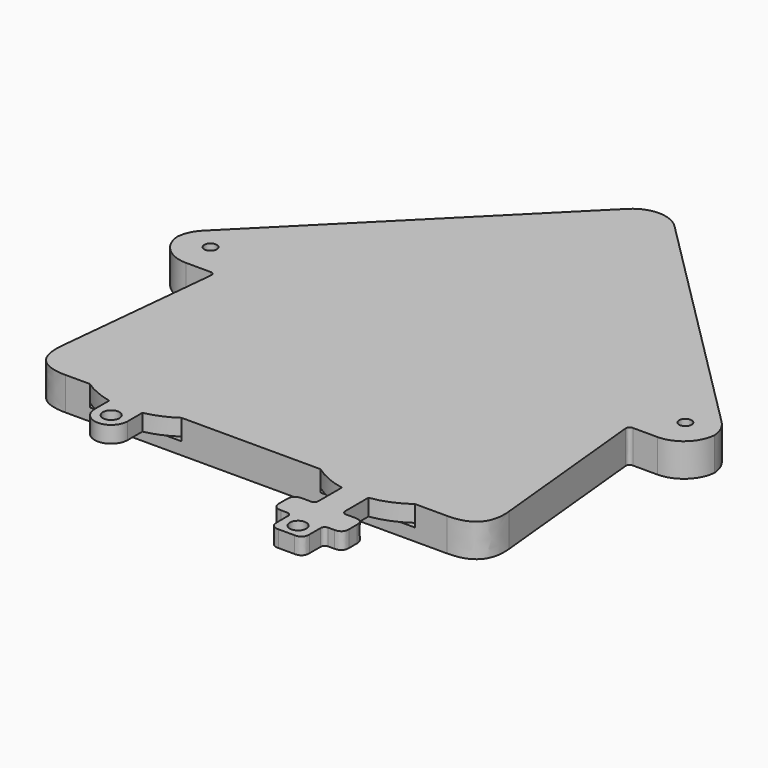
from build123d import *

# Parameters (mm, degrees)
F1_DEPTH    = 8
F2_T1_DEPTH = 24.5685424949
F2_T3_DEPTH = 48
F3_T1_DEPTH = 8
F4_T1_DEPTH = 52.1995024845
F5_R        = 13.5
F5_R_2      = 2
F6_DEPTH    = 5
F7_DEPTH    = 4
F8_T1_DEPTH = 14
F9_R        = 1
F10_R       = 1.5
F11_DEPTH   = 25


# Not quite as in the source:
# - a fillet or chamfer that OpenCascade refuses, or shapes differently, is made with other operations: its cross-section is extruded or revolved along the edge and cut away or added


with BuildPart() as f1:
    # F0 (on Top) → F1 (new body)
    with BuildSketch(Plane.XY):
        Polygon((65, 0), (0, 65), (-65, 0), (-65, -10), (-50, -10), (-55, -60), (0, -60), (55, -60), (50, -10), (65, -10), align=None)
    extrude(amount=F1_DEPTH)

    # F2: fillet of radius 8 on 5 edges, made by hand

    # F2_s2 → F2_t1 (cut)
    with BuildSketch(Plane.XY.offset(-8.2842712475)):
        with BuildLine():
            ThreePointArc((-65, -3.313708499), (-64.3910362601, -0.2522410401), (-62.6568542495, 2.3431457505))
            Line((-62.6568542495, 2.3431457505), (-65, 0))
            Line((-65, 0), (-65, -3.313708499))
        make_face()
        with BuildLine():
            ThreePointArc((62.6568542495, 2.3431457505), (64.3910362601, -0.2522410401), (65, -3.313708499))
            Line((65, -3.313708499), (65, 0))
            Line((65, 0), (62.6568542495, 2.3431457505))
        make_face()
    extrude(amount=F2_T1_DEPTH, mode=Mode.SUBTRACT)

    # F2_s4 → F2_t3 (cut)
    with BuildSketch(Plane.XY.offset(-20)):
        with BuildLine():
            ThreePointArc((5.6568542495, 59.3431457505), (0, 61.686291501), (-5.6568542495, 59.3431457505))
            Line((-5.6568542495, 59.3431457505), (0, 65))
            Line((0, 65), (5.6568542495, 59.3431457505))
        make_face()
        with BuildLine():
            ThreePointArc((57, -10), (62.6568542495, -7.6568542495), (65, -2))
            Line((65, -2), (65, -10))
            Line((65, -10), (57, -10))
        make_face()
        with BuildLine():
            ThreePointArc((-57, -10), (-62.6568542495, -7.6568542495), (-65, -2))
            Line((-65, -2), (-65, -10))
            Line((-65, -10), (-57, -10))
        make_face()
    extrude(amount=F2_T3_DEPTH, mode=Mode.SUBTRACT)

    # F3: fillet of radius 1 on 2 edges, made by hand

    # F3_s2 → F3_t1 (join)
    with BuildSketch(Plane.XY):
        with BuildLine():
            add(Edge.make_bspline(
                [(51.1049875621, -10), (50, -10), (50.1099503719, -11.099503719)],
                knots=[0, 0, 0, 1, 1, 1], degree=2, weights=[1, 1, 1]))
            Line((50.1099503719, -11.099503719), (50, -10))
            Line((50, -10), (51.1049875621, -10))
        make_face()
        with BuildLine():
            add(Edge.make_bspline(
                [(-50.1099503719, -11.099503719), (-50, -10), (-51.1049875621, -10)],
                knots=[0, 0, 0, 1, 1, 1], degree=2, weights=[1, 1, 1]))
            Line((-51.1049875621, -10), (-50, -10))
            Line((-50, -10), (-50.1099503719, -11.099503719))
        make_face()
    extrude(amount=F3_T1_DEPTH)

    # F4: fillet of radius 8 on 2 edges, made by hand

    # F4_s2 → F4_t1 (cut)
    with BuildSketch(Plane.XY.offset(-22.0997512422)):
        with BuildLine():
            add(Edge.make_bspline(
                [(-46.1600995031, -60), (-55, -60), (-54.1203970248, -51.2039702478)],
                knots=[0, 0, 0, 1, 1, 1], degree=2, weights=[1, 1, 1]))
            Line((-54.1203970248, -51.2039702478), (-55, -60))
            Line((-55, -60), (-46.1600995031, -60))
        make_face()
        with BuildLine():
            add(Edge.make_bspline(
                [(54.1203970248, -51.2039702478), (55, -60), (46.1600995031, -60)],
                knots=[0, 0, 0, 1, 1, 1], degree=2, weights=[1, 1, 1]))
            Line((46.1600995031, -60), (55, -60))
            Line((55, -60), (54.1203970248, -51.2039702478))
        make_face()
    extrude(amount=F4_T1_DEPTH, mode=Mode.SUBTRACT)

    # F5 (on face) → F6 (cut)
    with BuildSketch(Plane.XY.offset(8)):
        with BuildLine():
            Line((-8.4674237296, -19.0932191908), (-17.8053588669, -28.0791480434))
            ThreePointArc((-17.8053588669, -28.0791480434), (-45.0974523982, -32.7464944514), (-40.2098223871, -60))
            Line((-40.2098223871, -60), (-18.0631891992, -60))
            ThreePointArc((-18.0631891992, -60), (-11.8712274348, -53.0133159845), (-9.6365057932, -43.9490916266))
            ThreePointArc((-9.6365057932, -43.9490916266), (-10.5536669898, -38.0390914567), (-13.2188752299, -32.6850320897))
            Line((-13.2188752299, -32.6850320897), (-4.2390260021, -24.0298833133))
            Line((-4.2390260021, -24.0298833133), (-4.2390260021, -29.9932191908))
            Line((-4.2390260021, -29.9932191908), (1.8609739979, -29.9932191908))
            Line((1.8609739979, -29.9932191908), (1.8609739979, -12.9932191908))
            Line((1.8609739979, -12.9932191908), (-15.1390260021, -12.9932191908))
            Line((-15.1390260021, -12.9932191908), (-15.1390260021, -19.0932191908))
            Line((-15.1390260021, -19.0932191908), (-8.4674237296, -19.0932191908))
        make_face()
        with Locations((-29.1365057932, -43.9490916266)):
            Circle(F5_R, mode=Mode.SUBTRACT)
        with BuildLine():
            Line((-18.0631891992, -60), (-40.2098223871, -60))
            ThreePointArc((-40.2098223871, -60), (-36.8140065496, -61.8741015885), (-33.1144459271, -63.039036422))
            Line((-33.1144459271, -63.039036422), (-33.1144459271, -67.4490812726))
            ThreePointArc((-33.1144459271, -67.4490812726), (-29.1144459271, -71.4490812726), (-25.1144459271, -67.4490812726))
            Line((-25.1144459271, -67.4490812726), (-25.1144459271, -63.0297895812))
            ThreePointArc((-25.1144459271, -63.0297895812), (-21.4382914649, -61.8652155421), (-18.0631891992, -60))
        make_face()
        with Locations((-29.1144459271, -67.4490812726)):
            Circle(F5_R_2, mode=Mode.SUBTRACT)
        with BuildLine():
            Line((38.4021761528, -60), (15.5300545524, -60))
            ThreePointArc((15.5300545524, -60), (19.2758562864, -62.1250310842), (23.3967523072, -63.3760321733))
            Line((23.3967523072, -63.3760321733), (23.3967523072, -71.4671202268))
            Line((23.3967523072, -71.4671202268), (18.1967523072, -71.4671202268))
            Line((18.1967523072, -71.4671202268), (18.1967523072, -77.7814015746))
            Line((18.1967523072, -77.7814015746), (22.6967523072, -77.7814015746))
            Line((22.6967523072, -77.7814015746), (22.6967523072, -84.1620080173))
            Line((22.6967523072, -84.1620080173), (30.5967523072, -84.1620080173))
            Line((30.5967523072, -84.1620080173), (30.5967523072, -77.7814015746))
            Line((30.5967523072, -77.7814015746), (35.0967523072, -77.7814015746))
            Line((35.0967523072, -77.7814015746), (35.0967523072, -71.4671202268))
            Line((35.0967523072, -71.4671202268), (29.8967523072, -71.4671202268))
            Line((29.8967523072, -71.4671202268), (29.8967523072, -63.48401191))
            ThreePointArc((29.8967523072, -63.48401191), (34.357670388, -62.2502940054), (38.4021761528, -60))
        make_face()
        with Locations((26.6467523072, -80.6736797094)):
            Circle(F5_R_2, mode=Mode.SUBTRACT)
        with BuildLine():
            ThreePointArc((7.4678010834, -43.9490916266), (9.5407945482, -52.9581017828), (15.5300545524, -60))
            Line((15.5300545524, -60), (38.4021761528, -60))
            ThreePointArc((38.4021761528, -60), (35.9470895566, -26.8967619578), (7.4678010834, -43.9490916266))
        make_face()
        with BuildLine():
            ThreePointArc((40.4661153526, -44.2054910373), (26.8379098659, -57.7048822588), (13.4685504114, -43.9490916266))
            ThreePointArc((13.4685504114, -43.9490916266), (27.0943208393, -30.7060998157), (40.4661153526, -44.2054910373))
        make_face(mode=Mode.SUBTRACT)
    extrude(amount=-F6_DEPTH, mode=Mode.SUBTRACT)

    # F5 (on face) → F7 (join)
    with BuildSketch(Plane.XY.offset(8)):
        with BuildLine():
            Line((-8.4674237296, -19.0932191908), (-17.8053588669, -28.0791480434))
            ThreePointArc((-17.8053588669, -28.0791480434), (-46.9989205625, -36.1270625672), (-33.1144459271, -63.039036422))
            Line((-33.1144459271, -63.039036422), (-33.1144459271, -67.4490812726))
            ThreePointArc((-33.1144459271, -67.4490812726), (-29.1144459271, -71.4490812726), (-25.1144459271, -67.4490812726))
            Line((-25.1144459271, -67.4490812726), (-25.1144459271, -63.0297895812))
            ThreePointArc((-25.1144459271, -63.0297895812), (-13.99252733, -56.2336313537), (-9.6365057932, -43.9490916266))
            ThreePointArc((-9.6365057932, -43.9490916266), (-10.5536669898, -38.0390914567), (-13.2188752299, -32.6850320897))
            Line((-13.2188752299, -32.6850320897), (-4.2390260021, -24.0298833133))
            Line((-4.2390260021, -24.0298833133), (-4.2390260021, -29.9932191908))
            Line((-4.2390260021, -29.9932191908), (1.8609739979, -29.9932191908))
            Line((1.8609739979, -29.9932191908), (1.8609739979, -12.9932191908))
            Line((1.8609739979, -12.9932191908), (-15.1390260021, -12.9932191908))
            Line((-15.1390260021, -12.9932191908), (-15.1390260021, -19.0932191908))
            Line((-15.1390260021, -19.0932191908), (-8.4674237296, -19.0932191908))
        make_face()
        with Locations((-29.1144459271, -67.4490812726)):
            Circle(F5_R_2, mode=Mode.SUBTRACT)
        with Locations((-29.1365057932, -43.9490916266)):
            Circle(F5_R, mode=Mode.SUBTRACT)
        with BuildLine():
            ThreePointArc((29.8967523072, -63.48401191), (39.7733500471, -29.500908776), (7.4678010834, -43.9490916266))
            ThreePointArc((7.4678010834, -43.9490916266), (11.8869595763, -56.5695138889), (23.3967523072, -63.3760321733))
            Line((23.3967523072, -63.3760321733), (23.3967523072, -71.4671202268))
            Line((23.3967523072, -71.4671202268), (18.1967523072, -71.4671202268))
            Line((18.1967523072, -71.4671202268), (18.1967523072, -77.7814015746))
            Line((18.1967523072, -77.7814015746), (22.6967523072, -77.7814015746))
            Line((22.6967523072, -77.7814015746), (22.6967523072, -84.1620080173))
            Line((22.6967523072, -84.1620080173), (30.5967523072, -84.1620080173))
            Line((30.5967523072, -84.1620080173), (30.5967523072, -77.7814015746))
            Line((30.5967523072, -77.7814015746), (35.0967523072, -77.7814015746))
            Line((35.0967523072, -77.7814015746), (35.0967523072, -71.4671202268))
            Line((35.0967523072, -71.4671202268), (29.8967523072, -71.4671202268))
            Line((29.8967523072, -71.4671202268), (29.8967523072, -63.48401191))
        make_face()
        with Locations((26.6467523072, -80.6736797094)):
            Circle(F5_R_2, mode=Mode.SUBTRACT)
        with BuildLine():
            ThreePointArc((40.4661153526, -44.2054910373), (26.8379098659, -57.7048822588), (13.4685504114, -43.9490916266))
            ThreePointArc((13.4685504114, -43.9490916266), (27.0943208393, -30.7060998157), (40.4661153526, -44.2054910373))
        make_face(mode=Mode.SUBTRACT)
    extrude(amount=-F7_DEPTH)

    # F8: fillet of radius 2 on 6 edges, made by hand

    # F8_s2 → F8_t1 (cut)
    with BuildSketch(Plane.XY.offset(-1)):
        with BuildLine():
            add(Edge.make_bspline(
                [(30.5967523072, -82.1620080173), (30.5967523072, -84.1620080173), (28.5967523072, -84.1620080173)],
                knots=[0, 0, 0, 1, 1, 1], degree=2, weights=[1, 1, 1]))
            Line((28.5967523072, -84.1620080173), (30.5967523072, -84.1620080173))
            Line((30.5967523072, -84.1620080173), (30.5967523072, -82.1620080173))
        make_face()
        with BuildLine():
            add(Edge.make_bspline(
                [(24.6967523072, -84.1620080173), (22.6967523072, -84.1620080173), (22.6967523072, -82.1620080173)],
                knots=[0, 0, 0, 1, 1, 1], degree=2, weights=[1, 1, 1]))
            Line((22.6967523072, -82.1620080173), (22.6967523072, -84.1620080173))
            Line((22.6967523072, -84.1620080173), (24.6967523072, -84.1620080173))
        make_face()
        with BuildLine():
            add(Edge.make_bspline(
                [(20.1967523072, -77.7814015746), (18.1967523072, -77.7814015746), (18.1967523072, -75.7814015746)],
                knots=[0, 0, 0, 1, 1, 1], degree=2, weights=[1, 1, 1]))
            Line((18.1967523072, -75.7814015746), (18.1967523072, -77.7814015746))
            Line((18.1967523072, -77.7814015746), (20.1967523072, -77.7814015746))
        make_face()
        with BuildLine():
            add(Edge.make_bspline(
                [(35.0967523072, -75.7814015746), (35.0967523072, -77.7814015746), (33.0967523072, -77.7814015746)],
                knots=[0, 0, 0, 1, 1, 1], degree=2, weights=[1, 1, 1]))
            Line((33.0967523072, -77.7814015746), (35.0967523072, -77.7814015746))
            Line((35.0967523072, -77.7814015746), (35.0967523072, -75.7814015746))
        make_face()
        with BuildLine():
            add(Edge.make_bspline(
                [(33.0967523072, -71.4671202268), (35.0967523072, -71.4671202268), (35.0967523072, -73.4671202268)],
                knots=[0, 0, 0, 1, 1, 1], degree=2, weights=[1, 1, 1]))
            Line((35.0967523072, -73.4671202268), (35.0967523072, -71.4671202268))
            Line((35.0967523072, -71.4671202268), (33.0967523072, -71.4671202268))
        make_face()
        with BuildLine():
            add(Edge.make_bspline(
                [(18.1967523072, -73.4671202268), (18.1967523072, -71.4671202268), (20.1967523072, -71.4671202268)],
                knots=[0, 0, 0, 1, 1, 1], degree=2, weights=[1, 1, 1]))
            Line((20.1967523072, -71.4671202268), (18.1967523072, -71.4671202268))
            Line((18.1967523072, -71.4671202268), (18.1967523072, -73.4671202268))
        make_face()
    extrude(amount=F8_T1_DEPTH, mode=Mode.SUBTRACT)

    # F9
    f9_edges = [f1.edges().sort_by_distance(p)[0] for p in [
        (23.396752, -71.46712, 6),
        (29.896752, -71.46712, 6),
        (30.596752, -77.781402, 6),
        (22.696752, -77.781402, 6),
    ]]
    fillet(f9_edges, radius=F9_R)

    # F10 (on face) → F11 (cut)
    with BuildSketch(Plane.XY.offset(8)):
        with Locations((-57.4082396924, -2.0584366284)):
            Circle(F10_R)
        with Locations((57.4082396924, -2.0584366284)):
            Circle(F10_R)
    extrude(amount=-F11_DEPTH, mode=Mode.SUBTRACT)


solid = f1.part
